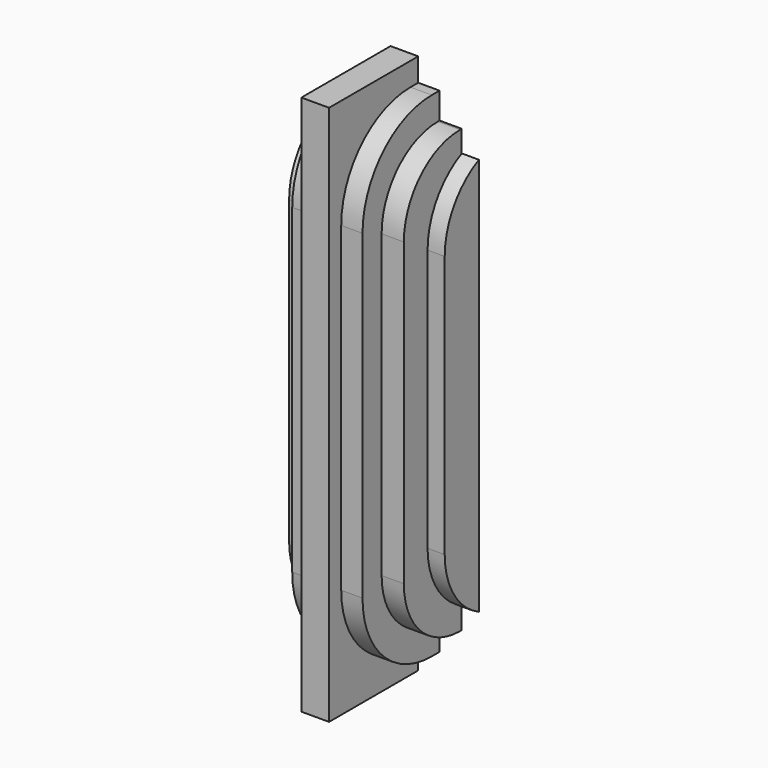
from build123d import *

# Parameters (mm, degrees)
F1_DEPTH      = 39.116
F2_DEPTH      = 33.782
F3_DEPTH      = 33.782
F4_DEPTH      = 25.4
F5_DEPTH      = 25.4
F0_W          = 6.0111228377
F0_H          = 69.8404787108
F6_DEPTH      = 14.986
F7_DEPTH      = 14.986
F8_T1_DEPTH   = 65.4734383573
F8_T6_DEPTH   = 124.9357538769
F10_R         = 24.6510518427
F11_R         = 24.6634
F12_R         = 30.3539071197
F14_T         = -2.54
F15_DEPTH     = 14.986
F16_T1_DEPTH  = 124.9268049826
F17_DEPTH     = 25.4
F18_R         = 24.6634
F19_DEPTH     = 33.782
F20_R         = 30.353
F21_DEPTH     = 39.116
F22_DEPTH     = 33.782
F23_DEPTH     = 25.4
F24_DEPTH     = 14.986
F25_T1_DEPTH  = 65.4689639101
F25_T6_DEPTH  = 124.9268049826
F26_R         = 24.6634
F27_R         = 30.353
F28_T         = 2.54
F28_T3_DEPTH  = 5.8166
F28_T5_DEPTH  = 110.6669781681
F28_T7_DEPTH  = 5.8289481573
F28_T9_DEPTH  = 8.509
F28_T11_DEPTH = 117.7830652202
F28_T13_DEPTH = 8.5080928803
F28_T15_DEPTH = 110.6546300108
F28_T17_DEPTH = 97.1928947849
F28_T19_DEPTH = 41.656
F28_T21_DEPTH = 9.7208591178
F28_T23_DEPTH = 10.414
F28_T25_DEPTH = 94.8683656752
F28_T27_DEPTH = 58.8910790502
F28_T29_DEPTH = 13.462
F28_T31_DEPTH = 55.3396631627
F28_T33_DEPTH = 15.494
F28_T35_DEPTH = 17.526
F28_T37_DEPTH = 48.595552503
F28_T39_DEPTH = 12.5542403813
F28_T41_DEPTH = 12.8764020893
F28_T43_DEPTH = 11.0911228377
F28_T45_DEPTH = 11.0911228377
F28_T47_DEPTH = 12.8764020893
F28_T49_DEPTH = 12.5542403813
F28_T51_DEPTH = 55.3273150054
F28_T54_ANGLE = 90.000000001
F28_T56_ANGLE = 90.000000001
F28_T58_ANGLE = 90.000000001
F28_T60_ANGLE = 90.000000001
F28_T62_ANGLE = 90.000000001
F28_T64_ANGLE = 90.000000001
F28_T66_ANGLE = 90.000000001
F28_T68_ANGLE = 90.000000001
F28_T70_ANGLE = 64.4309058664
F28_T72_ANGLE = 64.4270166015
F28_T74_ANGLE = 64.4309058664
F28_T76_ANGLE = 64.4270166015
F28_T78_ANGLE = 90.000000001
F28_T80_ANGLE = 90.000000001
F28_T82_ANGLE = 61.4663888849
F28_T84_ANGLE = 61.4663888848
F28_T86_ANGLE = 90.000000001
F28_T88_ANGLE = 90.000000001
F30_DEPTH     = 81.788


# Not quite as in the source:
# - a fillet or chamfer that OpenCascade refuses, or shapes differently, is made with other operations: its cross-section is extruded or revolved along the edge and cut away or added
# - two fillets or chamfers of one size are made in one step
# - a feature of the source that left no trace in its solid (it failed there, or was rolled back) is left out
# - a shell that OpenCascade refuses in one call is made with other operations: the cavity is built on its own and cut out


with BuildPart() as f1:
    # F0 (on Front) → F1 (new body)
    with BuildSketch(Plane.XZ):
        Polygon((4.8604295589, 33.4735736251), (0, 33.4735736251), (-4.8604295589, 33.4735736251), (-4.8604295589, 25.3101941198), (-4.8604295589, -61.3947920501), (4.8604295589, -61.3947920501), (4.8604295589, 25.3101941198), align=None)
    extrude(amount=F1_DEPTH)

    # F0 (on Front) → F2 (join)
    with BuildSketch(Plane.XZ):
        Polygon((-4.8604295589, -61.3947920501), (-4.8604295589, 25.3101941198), (-12.3346699402, 25.3101941198), (-12.3346699402, 16.0559229553), (-12.3346699402, -61.3947920501), align=None)
    extrude(amount=F2_DEPTH)

    # F0 (on Front) → F3 (join)
    with BuildSketch(Plane.XZ):
        Polygon((12.3346699402, 25.3101941198), (4.8604295589, 25.3101941198), (4.8604295589, -61.3947920501), (12.3346699402, -61.3947920501), (12.3346699402, 16.0559229553), align=None)
    extrude(amount=F3_DEPTH)

    # F0 (on Front) → F4 (join)
    with BuildSketch(Plane.XZ):
        Polygon((-20.1310720295, -61.3947920501), (-12.3346699402, -61.3947920501), (-12.3346699402, 16.0559229553), (-20.1310720295, 16.0559229553), (-20.1310720295, 8.4456866607), align=None)
    extrude(amount=F4_DEPTH)

    # F0 (on Front) → F5 (join)
    with BuildSketch(Plane.XZ):
        Polygon((12.3346699402, 16.0559229553), (12.3346699402, -61.3947920501), (20.1310720295, -61.3947920501), (20.1310720295, 8.4456866607), (20.1310720295, 16.0559229553), align=None)
    extrude(amount=F5_DEPTH)

    # F0 (on Front) → F6 (join)
    with BuildSketch(Plane.XZ):
        with Locations((-23.1366334483, -26.4745526947)):
            Rectangle(F0_W, F0_H)
    extrude(amount=F6_DEPTH)

    # F0 (on Front) → F7 (join)
    with BuildSketch(Plane.XZ):
        with Locations((23.1366334483, -26.4745526947)):
            Rectangle(F0_W, F0_H)
    extrude(amount=F7_DEPTH)

    # F8: fillet of radius 26.3680405282 on 1 edges, made by hand

    # F8_s2 → F8_t1 (cut)
    with BuildSketch(Plane.YZ.offset(20.1310720295)):
        with BuildLine():
            ThreePointArc((-14.986, -15.3392395471), (-10.9271018493, -1.2830762129), (0, 8.4456866607))
            Line((0, 8.4456866607), (-0.2276408106, 8.9213851849))
            ThreePointArc((-0.2276408106, 8.9213851849), (-7.493, 8.9730474713), (-14.986, 8.9730474713))
            Line((-14.986, 8.9730474713), (-15.5133608106, 8.4456866607))
            Line((-15.5133608106, 8.4456866607), (-15.5133608106, -15.3392395471))
            Line((-15.5133608106, -15.3392395471), (-14.986, -15.3392395471))
        make_face()
    extrude(amount=F8_T1_DEPTH, mode=Mode.SUBTRACT)


with BuildPart() as f8_tool4:
    # F8_s5 → F8_t6 (new body)
    with BuildSketch(Plane.YZ.offset(85.6045103867)):
        with BuildLine():
            ThreePointArc((-14.986, -15.3392395471), (-10.9271018493, -1.2830762129), (0, 8.4456866607))
            Line((0, 8.4456866607), (-0.2276408106, 8.9213851849))
            ThreePointArc((-0.2276408106, 8.9213851849), (-7.493, 8.9730474713), (-14.986, 8.9730474713))
            Line((-14.986, 8.9730474713), (-15.5133608106, 8.4456866607))
            Line((-15.5133608106, 8.4456866607), (-15.5133608106, -15.3392395471))
            Line((-15.5133608106, -15.3392395471), (-14.986, -15.3392395471))
        make_face()
    extrude(amount=-F8_T6_DEPTH)

    split(bisect_by=Plane.YZ.offset(-20.1310720295), keep=Keep.BOTTOM)


with BuildPart() as f1_1:
    add(f1.part)

    # F8_t3: cut F8_tool4
    add(f8_tool4.part, mode=Mode.SUBTRACT)

    # F10
    f10_edges = [f1_1.edges().sort_by_distance(p)[0] for p in [
        (16.232871, -25.4, 16.055923),
    ]]
    fillet(f10_edges, radius=F10_R)

    # F11
    f11_edges = [f1_1.edges().sort_by_distance(p)[0] for p in [
        (-16.232871, -25.4, 16.055923),
    ]]
    fillet(f11_edges, radius=F11_R)

    # F12
    f12_edges = [f1_1.edges().sort_by_distance(p)[0] for p in [
        (-8.59755, -33.782, 25.310194),
        (8.59755, -33.782, 25.310194),
    ]]
    fillet(f12_edges, radius=F12_R)

    # F14
    f14_openings = [f1_1.faces().sort_by_distance(p)[0] for p in [
        (0, 0, -20.12968),
    ]]
    offset(amount=F14_T, openings=f14_openings, kind=Kind.INTERSECTION)

    # F0 (on Front) → F15 (join)
    with BuildSketch(Plane.XZ):
        with Locations((-23.1366334483, -96.3150314055)):
            Rectangle(F0_W, F0_H)
    extrude(amount=F15_DEPTH)

    # F16: fillet of radius 26.3652 on 1 edges, made by hand

    # F16_s2 → F16_t1 (cut)
    with BuildSketch(Plane.YZ.offset(-85.6000359396)):
        with BuildLine():
            ThreePointArc((-14.986, -107.452134332), (-10.9270620679, -121.5075405374), (0, -131.235270761))
            Line((0, -131.235270761), (-14.986, -131.235270761))
            Line((-14.986, -131.235270761), (-14.986, -107.452134332))
        make_face()
    extrude(amount=F16_T1_DEPTH, mode=Mode.SUBTRACT)

    # F0 (on Front) → F17 (join)
    with BuildSketch(Plane.XZ):
        Polygon((-12.3346699402, -138.8455070555), (-12.3346699402, -61.3947920501), (-20.1310720295, -61.3947920501), (-20.1310720295, -131.235270761), (-20.1310720295, -138.8455070555), align=None)
    extrude(amount=F17_DEPTH)

    # F18
    f18_edges = [f1_1.edges().sort_by_distance(p)[0] for p in [
        (-16.232871, -25.4, -138.845507),
    ]]
    fillet(f18_edges, radius=F18_R)

    # F0 (on Front) → F19 (join)
    with BuildSketch(Plane.XZ):
        Polygon((-4.8604295589, -148.0997782201), (-4.8604295589, -61.3947920501), (-12.3346699402, -61.3947920501), (-12.3346699402, -138.8455070555), (-12.3346699402, -148.0997782201), align=None)
    extrude(amount=F19_DEPTH)

    # F20
    f20_edges = [f1_1.edges().sort_by_distance(p)[0] for p in [
        (-8.59755, -33.782, -148.099778),
    ]]
    fillet(f20_edges, radius=F20_R)

    # F0 (on Front) → F21 (join)
    with BuildSketch(Plane.XZ):
        Polygon((4.8604295589, -61.3947920501), (-4.8604295589, -61.3947920501), (-4.8604295589, -148.0997782201), (-4.8604295589, -156.2631577253), (0, -156.2631577253), (4.8604295589, -156.2631577253), (4.8604295589, -148.0997782201), align=None)
    extrude(amount=F21_DEPTH)

    # F0 (on Front) → F22 (join)
    with BuildSketch(Plane.XZ):
        Polygon((12.3346699402, -61.3947920501), (4.8604295589, -61.3947920501), (4.8604295589, -148.0997782201), (12.3346699402, -148.0997782201), (12.3346699402, -138.8455070555), align=None)
    extrude(amount=F22_DEPTH)

    # F0 (on Front) → F23 (join)
    with BuildSketch(Plane.XZ):
        Polygon((20.1310720295, -61.3947920501), (12.3346699402, -61.3947920501), (12.3346699402, -138.8455070555), (20.1310720295, -138.8455070555), (20.1310720295, -131.235270761), align=None)
    extrude(amount=F23_DEPTH)

    # F0 (on Front) → F24 (join)
    with BuildSketch(Plane.XZ):
        with Locations((23.1366334483, -96.3150314055)):
            Rectangle(F0_W, F0_H)
    extrude(amount=F24_DEPTH)

    # F25: fillet of radius 26.3652 on 1 edges, made by hand

    # F25_s2 → F25_t1 (cut)
    with BuildSketch(Plane.YZ.offset(20.1310720295)):
        with BuildLine():
            ThreePointArc((0, -131.235270761), (-10.9270620679, -121.5075405374), (-14.986, -107.452134332))
            Line((-14.986, -107.452134332), (-15.513304, -107.452134332))
            Line((-15.513304, -107.452134332), (-15.513304, -131.235270761))
            Line((-15.513304, -131.235270761), (-14.986, -131.762574761))
            ThreePointArc((-14.986, -131.762574761), (-7.493, -131.762574761), (-0.227584, -131.7109334895))
            Line((-0.227584, -131.7109334895), (0, -131.235270761))
        make_face()
    extrude(amount=F25_T1_DEPTH, mode=Mode.SUBTRACT)


with BuildPart() as f25_tool4:
    # F25_s5 → F25_t6 (new body)
    with BuildSketch(Plane.YZ.offset(-39.326769043)):
        with BuildLine():
            ThreePointArc((0, -131.235270761), (-10.9270620679, -121.5075405374), (-14.986, -107.452134332))
            Line((-14.986, -107.452134332), (-15.513304, -107.452134332))
            Line((-15.513304, -107.452134332), (-15.513304, -131.235270761))
            Line((-15.513304, -131.235270761), (-14.986, -131.762574761))
            ThreePointArc((-14.986, -131.762574761), (-7.493, -131.762574761), (-0.227584, -131.7109334895))
            Line((-0.227584, -131.7109334895), (0, -131.235270761))
        make_face()
    extrude(amount=F25_T6_DEPTH)

    split(bisect_by=Plane.YZ.offset(-20.1310720295), keep=Keep.BOTTOM)


with BuildPart() as f1_2:
    add(f1_1.part)

    # F25_t3: cut F25_tool4
    add(f25_tool4.part, mode=Mode.SUBTRACT)

    # F26
    f26_edges = [f1_2.edges().sort_by_distance(p)[0] for p in [
        (16.232871, -25.4, -138.845507),
    ]]
    fillet(f26_edges, radius=F26_R)

    # F27
    f27_edges = [f1_2.edges().sort_by_distance(p)[0] for p in [
        (8.59755, -33.782, -148.099778),
    ]]
    fillet(f27_edges, radius=F27_R)

    # F28: shell of thickness 2.54, made by hand


with BuildPart() as f28_core1:
    # F28_t2: copy of F1
    add(f1_2.part)

    # the walls: a layer under each face that stays
    f28_faces = [f28_core1.faces().sort_by_distance(p)[0] for p in [
        (12.3346699402, -28.1516666667, -119.1981161634),
        (8.5975497495, -1.7145, -148.0997782201),
        (8.5975497495, -24.8918121294, -139.2095903494),
        (8.5975497495, -33.782, -61.39524561),
        (16.2328709848, -0.3683, -138.8455070555),
        (8.5975497495, -24.8915464401, 16.41974056),
        (16.2328709848, -18.1762573871, -131.6217644426),
        (8.5975497495, -1.7140464401, 25.3101941198),
        (16.2328709848, -25.4, -61.3886179715),
        (16.2328709848, -18.1798740787, 8.8357970339),
        (16.2328709848, -0.3744740787, 16.0559229553),
        (4.8604295589, -36.322, -142.7105340574),
        (0, -19.558, 33.4735736251),
        (-4.8604295589, -36.322, 19.9209499572),
        (-8.5975497495, -1.7140464401, 25.3101941198),
        (-12.3346699402, -28.1516666667, -3.5914679368),
        (-16.2328709848, -0.3683, 16.0559229553),
        (-20.1310720295, -21.1666666667, -9.7609820465),
        (-23.1366334483, -10.9271018493, -1.2830762129),
        (-26.1421948671, -7.493, -61.3947920501),
        (-23.1366334483, -10.9270620679, -121.5075405375),
        (-16.2328709848, -0.3683, -138.8455070555),
        (-8.5975497495, -1.7145, -148.0997782201),
        (0, -19.558, -156.2631577253),
        (20.1310720295, -21.1666666667, -113.0286020537),
        (23.1366334483, -10.9270620679, -121.5075405375),
        (26.1421948671, -7.493, -61.3947920501),
        (23.1366334483, -10.9271018493, -1.2830762129),
        (0, -18.288, 30.9335736251),
        (2.3204295589, -30.48, 15.9688460126),
        (6.0575497495, -1.7140464401, 22.7701941198),
        (9.7946699402, -26.035, -45.2506276885),
        (13.6928709848, -0.3744740787, 13.5159229553),
        (17.5910720295, -19.05, -46.7930062159),
        (20.5966334483, -9.0995028513, -3.1621341354),
        (23.6021948671, -6.223, -26.6301076015),
        (0, -18.288, -58.8547920501),
        (-23.6021948671, -6.223, -26.6301076015),
        (-20.5966334483, -9.0995028513, -3.1621341354),
        (-17.5910720295, -19.05, 1.454137121),
        (-13.6928709848, -0.3683, 13.5159229553),
        (-9.7946699402, -26.035, 9.1660297582),
        (-6.0575497495, -1.7140464401, 22.7701941198),
        (-2.3204295589, -30.48, 15.9688460126),
        (0, -39.116, -61.3947920501),
        (-8.5975497495, -33.782, -61.39524561),
        (-8.5975497495, -24.8915464401, 16.41974056),
        (-8.5975497495, -24.8918121294, -139.2095903494),
        (-16.2328709848, -18.1762573871, -131.6217644426),
        (-16.2328709848, -18.1762573871, 8.8321803424),
        (-16.2328709848, -25.4, -61.3947920501),
        (-23.1366334483, -14.986, -61.3956869396),
        (23.1366334483, -14.986, -61.3956869395),
        (0, -36.576, -13.9606092125),
        (6.0575497495, -31.242, -31.949252525),
        (6.0575497495, -23.0954952159, 14.6236893357),
        (13.6928709848, -16.3838228544, 7.0397458097),
        (13.6928709848, -22.86, -33.7249604688),
        (20.5966334483, -12.446, -37.0970157986),
        (-20.5966334483, -12.446, -37.0970157986),
        (-13.6928709848, -22.86, -33.7311345474),
        (-6.0575497495, -31.242, -31.949252525),
        (-13.6928709848, -16.3802061629, 7.0361291182),
        (-6.0575497495, -23.0954952159, 14.6236893357),
    ]]
    thicken(f28_faces, amount=-F28_T, mode=Mode.SUBTRACT)

    # F28_s4 → F28_t3 (cut)
    with BuildSketch(Plane.XZ.offset(-2.54)):
        Polygon((12.3600699402, -138.8709070555), (9.7946699402, -138.8455070555), (9.7946699402, -136.3055070555), (12.3346699402, -136.3055070555), align=None)
        Polygon((-12.3600699402, -138.8709070555), (-9.7946699402, -138.8455070555), (-9.7946699402, -136.3055070555), (-12.3346699402, -136.3055070555), align=None)
        Polygon((-12.3600699402, 16.0813229553), (-9.7946699402, 16.0559229553), (-9.7946699402, 13.5159229553), (-12.3346699402, 13.5159229553), align=None)
        Polygon((-17.5656720295, 13.4905229553), (-20.1310720295, 13.5159229553), (-20.1310720295, 16.0559229553), (-17.5910720295, 16.0559229553), align=None)
    extrude(amount=F28_T3_DEPTH, mode=Mode.SUBTRACT)

    # F28_s6 → F28_t5 (cut)
    with BuildSketch(Plane.XY.offset(-116.7221070555)):
        Polygon((12.3600699402, -25.4254), (9.7946699402, -25.4), (9.7946699402, -22.86), (12.3346699402, -22.86), align=None)
    extrude(amount=F28_T5_DEPTH, mode=Mode.SUBTRACT)

    # F28_s8 → F28_t7 (cut)
    with BuildSketch(Plane.XZ.offset(-2.54)):
        Polygon((12.3600699402, 16.0813229553), (9.7946699402, 16.0559229553), (9.7946699402, 13.5159229553), (12.3346699402, 13.5159229553), align=None)
        Polygon((17.5656720295, 13.4905229553), (17.5910720295, 16.0559229553), (20.1310720295, 16.0559229553), (20.1310720295, 13.5159229553), align=None)
    extrude(amount=F28_T7_DEPTH, mode=Mode.SUBTRACT)

    # F28_s10 → F28_t9 (cut)
    with BuildSketch(Plane.XZ.offset(-2.54)):
        Polygon((4.8858295589, -148.1251782201), (4.8604295589, -145.5597782201), (2.3204295589, -145.5597782201), (2.3204295589, -148.0997782201), align=None)
        Polygon((-4.8858295589, -148.1251782201), (-2.3204295589, -148.0997782201), (-2.3204295589, -145.5597782201), (-4.8604295589, -145.5597782201), align=None)
    extrude(amount=F28_T9_DEPTH, mode=Mode.SUBTRACT)

    # F28_s12 → F28_t11 (cut)
    with BuildSketch(Plane.XY.offset(-120.2867782201)):
        Polygon((4.8858295589, -33.8074), (4.8604295589, -31.242), (2.3204295589, -31.242), (2.3204295589, -33.782), align=None)
        Polygon((-4.8858295589, -33.8074), (-2.3204295589, -33.782), (-2.3204295589, -31.242), (-4.8604295589, -31.242), align=None)
    extrude(amount=F28_T11_DEPTH, mode=Mode.SUBTRACT)

    # F28_s14 → F28_t13 (cut)
    with BuildSketch(Plane.XZ.offset(-2.54)):
        Polygon((4.8858295589, 25.3355941198), (4.8604295589, 22.7701941198), (2.3204295589, 22.7701941198), (2.3204295589, 25.3101941198), align=None)
        Polygon((-4.8858295589, 25.3355941198), (-2.3204295589, 25.3101941198), (-2.3204295589, 22.7701941198), (-4.8604295589, 22.7701941198), align=None)
        Polygon((9.7692699402, 22.7447941198), (9.7946699402, 25.3101941198), (12.3346699402, 25.3101941198), (12.3346699402, 22.7701941198), align=None)
        Polygon((-9.7692699402, 22.7447941198), (-12.3346699402, 22.7701941198), (-12.3346699402, 25.3101941198), (-9.7946699402, 25.3101941198), align=None)
    extrude(amount=F28_T13_DEPTH, mode=Mode.SUBTRACT)

    # F28_s16 → F28_t15 (cut)
    with BuildSketch(Plane.XY.offset(-116.7221070555)):
        Polygon((-12.3600699402, -25.4254), (-9.7946699402, -25.4), (-9.7946699402, -22.86), (-12.3346699402, -22.86), align=None)
    extrude(amount=F28_T15_DEPTH, mode=Mode.SUBTRACT)

    # F28_s18 → F28_t17 (cut)
    with BuildSketch(Plane.XY.offset(-109.992134332)):
        Polygon((-20.1564720295, -15.0114), (-17.5910720295, -14.986), (-17.5910720295, -12.446), (-20.1310720295, -12.446), align=None)
        Polygon((20.1564720295, -15.0114), (17.5910720295, -14.986), (17.5910720295, -12.446), (20.1310720295, -12.446), align=None)
    extrude(amount=F28_T17_DEPTH, mode=Mode.SUBTRACT)

    # F28_s20 → F28_t19 (cut)
    with BuildSketch(Plane.XZ.offset(-2.54)):
        Polygon((2.2950295589, 30.9081736251), (2.3204295589, 33.4735736251), (4.8604295589, 33.4735736251), (4.8604295589, 30.9335736251), align=None)
        Polygon((-2.2950295589, 30.9081736251), (-2.3204295589, 33.4735736251), (-4.8604295589, 33.4735736251), (-4.8604295589, 30.9335736251), align=None)
    extrude(amount=F28_T19_DEPTH, mode=Mode.SUBTRACT)

    # F28_s22 → F28_t21 (cut)
    with BuildSketch(Plane.YZ.offset(-4.8604295589)):
        Polygon((-36.5506, 30.9081736251), (-36.576, 33.4735736251), (-39.116, 33.4735736251), (-39.116, 30.9335736251), align=None)
        Polygon((-36.5506, -58.8293920501), (-36.576, -61.3947920501), (-39.116, -61.3947920501), (-39.116, -58.8547920501), align=None)
    extrude(amount=F28_T21_DEPTH, mode=Mode.SUBTRACT)

    # F28_s24 → F28_t23 (cut)
    with BuildSketch(Plane.XZ.offset(28.702)):
        Polygon((2.2950295589, -58.8293920501), (4.8604295589, -58.8547920501), (4.8604295589, -61.3947920501), (2.3204295589, -61.3947920501), align=None)
        Polygon((-2.2950295589, -58.8293920501), (-2.3204295589, -61.3947920501), (-4.8604295589, -61.3947920501), (-4.8604295589, -58.8547920501), align=None)
    extrude(amount=F28_T23_DEPTH, mode=Mode.SUBTRACT)

    # F28_s26 → F28_t25 (cut)
    with BuildSketch(Plane.XY.offset(-61.3947920501)):
        Polygon((2.2950295589, -36.5506), (4.8604295589, -36.576), (4.8604295589, -39.116), (2.3204295589, -39.116), align=None)
        Polygon((-2.2950295589, -36.5506), (-4.8604295589, -36.576), (-4.8604295589, -39.116), (-2.3204295589, -39.116), align=None)
    extrude(amount=F28_T25_DEPTH, mode=Mode.SUBTRACT)

    # F28_s28 → F28_t27 (cut)
    with BuildSketch(Plane.XY.offset(-61.3947920501)):
        Polygon((9.7692699402, -31.2166), (12.3346699402, -31.242), (12.3346699402, -33.782), (9.7946699402, -33.782), align=None)
        Polygon((-9.7692699402, -31.2166), (-12.3346699402, -31.242), (-12.3346699402, -33.782), (-9.7946699402, -33.782), align=None)
    extrude(amount=F28_T27_DEPTH, mode=Mode.SUBTRACT)

    # F28_s30 → F28_t29 (cut)
    with BuildSketch(Plane.XZ.offset(20.32)):
        Polygon((9.7692699402, -58.8293920501), (12.3346699402, -58.8547920501), (12.3346699402, -61.3947920501), (9.7946699402, -61.3947920501), align=None)
        Polygon((-9.7692699402, -58.8293920501), (-9.7946699402, -61.3947920501), (-12.3346699402, -61.3947920501), (-12.3346699402, -58.8547920501), align=None)
    extrude(amount=F28_T29_DEPTH, mode=Mode.SUBTRACT)

    # F28_s32 → F28_t31 (cut)
    with BuildSketch(Plane.XY.offset(-61.3947920501)):
        Polygon((17.5656720295, -22.8346), (20.1310720295, -22.86), (20.1310720295, -25.4), (17.5910720295, -25.4), align=None)
    extrude(amount=F28_T31_DEPTH, mode=Mode.SUBTRACT)

    # F28_s34 → F28_t33 (cut)
    with BuildSketch(Plane.XZ.offset(9.906)):
        Polygon((17.5656720295, -58.8293920501), (20.1310720295, -58.8547920501), (20.1310720295, -61.3947920501), (17.5910720295, -61.3947920501), align=None)
        Polygon((-17.5656720295, -58.8293920501), (-17.5910720295, -61.3947920501), (-20.1310720295, -61.3947920501), (-20.1310720295, -58.8547920501), align=None)
    extrude(amount=F28_T33_DEPTH, mode=Mode.SUBTRACT)

    # F28_s36 → F28_t35 (cut)
    with BuildSketch(Plane.XZ.offset(-2.54)):
        Polygon((23.5767948671, -58.8293920501), (26.1421948671, -58.8547920501), (26.1421948671, -61.3947920501), (23.6021948671, -61.3947920501), align=None)
        Polygon((-23.5767948671, -58.8293920501), (-23.6021948671, -61.3947920501), (-26.1421948671, -61.3947920501), (-26.1421948671, -58.8547920501), align=None)
    extrude(amount=F28_T35_DEPTH, mode=Mode.SUBTRACT)

    # F28_s38 → F28_t37 (cut)
    with BuildSketch(Plane.XY.offset(-61.3947920501)):
        Polygon((23.5767948671, -12.4206), (26.1421948671, -12.446), (26.1421948671, -14.986), (23.6021948671, -14.986), align=None)
        Polygon((-23.5767948671, -12.4206), (-26.1421948671, -12.446), (-26.1421948671, -14.986), (-23.6021948671, -14.986), align=None)
    extrude(amount=F28_T37_DEPTH, mode=Mode.SUBTRACT)

    # F28_s40 → F28_t39 (cut)
    with BuildSketch(Plane.YZ.offset(-0.2195704411)):
        Polygon((-31.2166, -58.8293920501), (-31.242, -61.3947920501), (-33.782, -61.3947920501), (-33.782, -58.8547920501), align=None)
    extrude(amount=F28_T39_DEPTH, mode=Mode.SUBTRACT)

    # F28_s42 → F28_t41 (cut)
    with BuildSketch(Plane.YZ.offset(7.2546699402)):
        Polygon((-22.8346, -58.8293920501), (-22.86, -61.3947920501), (-25.4, -61.3947920501), (-25.4, -58.8547920501), align=None)
    extrude(amount=F28_T41_DEPTH, mode=Mode.SUBTRACT)

    # F28_s44 → F28_t43 (cut)
    with BuildSketch(Plane.YZ.offset(15.0510720295)):
        Polygon((-12.4206, -58.8293920501), (-12.446, -61.3947920501), (-14.986, -61.3947920501), (-14.986, -58.8547920501), align=None)
    extrude(amount=F28_T43_DEPTH, mode=Mode.SUBTRACT)

    # F28_s46 → F28_t45 (cut)
    with BuildSketch(Plane.YZ.offset(-26.1421948671)):
        Polygon((-12.4206, -58.8293920501), (-12.446, -61.3947920501), (-14.986, -61.3947920501), (-14.986, -58.8547920501), align=None)
    extrude(amount=F28_T45_DEPTH, mode=Mode.SUBTRACT)

    # F28_s48 → F28_t47 (cut)
    with BuildSketch(Plane.YZ.offset(-20.1310720295)):
        Polygon((-22.8346, -58.8293920501), (-22.86, -61.3947920501), (-25.4, -61.3947920501), (-25.4, -58.8547920501), align=None)
    extrude(amount=F28_T47_DEPTH, mode=Mode.SUBTRACT)

    # F28_s50 → F28_t49 (cut)
    with BuildSketch(Plane.YZ.offset(-12.3346699402)):
        Polygon((-31.2166, -58.8293920501), (-31.242, -61.3947920501), (-33.782, -61.3947920501), (-33.782, -58.8547920501), align=None)
    extrude(amount=F28_T49_DEPTH, mode=Mode.SUBTRACT)

    # F28_s52 → F28_t51 (cut)
    with BuildSketch(Plane.XY.offset(-61.3947920501)):
        Polygon((-17.5656720295, -22.8346), (-20.1310720295, -22.86), (-20.1310720295, -25.4), (-17.5910720295, -25.4), align=None)
    extrude(amount=F28_T51_DEPTH, mode=Mode.SUBTRACT)

    # F28_s53 → F28_t54 (revolve, cut)
    with BuildSketch(Plane.XZ.offset(0.7366)):
        Polygon((12.3600699402, -138.8709070555), (9.7946699402, -138.8455070555), (9.7946699402, -136.3055070555), (12.3346699402, -136.3055070555), align=None)
    revolve(axis=Axis((12.3346699402, -0.7366, -114.1821070555), (-1, 0, 0)), revolution_arc=F28_T54_ANGLE, mode=Mode.SUBTRACT)

    # F28_s55 → F28_t56 (revolve, cut)
    with BuildSketch(Plane.XZ.offset(0.7489481573)):
        Polygon((12.3600699402, 16.0813229553), (9.7946699402, 16.0559229553), (9.7946699402, 13.5159229553), (12.3346699402, 13.5159229553), align=None)
    revolve(axis=Axis((12.3346699402, -0.7489481573, -8.5951288874), (1, 0, 0)), revolution_arc=F28_T56_ANGLE, mode=Mode.SUBTRACT)

    # F28_s57 → F28_t58 (revolve, cut)
    with BuildSketch(Plane.XZ.offset(3.429)):
        Polygon((4.8858295589, -148.1251782201), (4.8604295589, -145.5597782201), (2.3204295589, -145.5597782201), (2.3204295589, -148.0997782201), align=None)
    revolve(axis=Axis((4.8604295589, -3.429, -117.7467782201), (-1, 0, 0)), revolution_arc=F28_T58_ANGLE, mode=Mode.SUBTRACT)

    # F28_s59 → F28_t60 (revolve, cut)
    with BuildSketch(Plane.XZ.offset(3.4280928803)):
        Polygon((4.8858295589, 25.3355941198), (4.8604295589, 22.7701941198), (2.3204295589, 22.7701941198), (2.3204295589, 25.3101941198), align=None)
    revolve(axis=Axis((4.8604295589, -3.4280928803, -5.0437129999), (1, 0, 0)), revolution_arc=F28_T60_ANGLE, mode=Mode.SUBTRACT)

    # F28_s61 → F28_t62 (revolve, cut)
    with BuildSketch(Plane.XZ.offset(3.4280928803)):
        Polygon((-4.8858295589, 25.3355941198), (-2.3204295589, 25.3101941198), (-2.3204295589, 22.7701941198), (-4.8604295589, 22.7701941198), align=None)
    revolve(axis=Axis((-4.8604295589, -3.4280928803, -5.0437129999), (1, 0, 0)), revolution_arc=F28_T62_ANGLE, mode=Mode.SUBTRACT)

    # F28_s63 → F28_t64 (revolve, cut)
    with BuildSketch(Plane.XY.offset(-117.7467782201)):
        Polygon((-4.8858295589, -33.8074), (-2.3204295589, -33.782), (-2.3204295589, -31.242), (-4.8604295589, -31.242), align=None)
    revolve(axis=Axis((-4.8604295589, -3.429, -117.7467782201), (1, 0, 0)), revolution_arc=F28_T64_ANGLE, mode=Mode.SUBTRACT)

    # F28_s65 → F28_t66 (revolve, cut)
    with BuildSketch(Plane.XY.offset(-114.1821070555)):
        Polygon((-12.3600699402, -25.4254), (-9.7946699402, -25.4), (-9.7946699402, -22.86), (-12.3346699402, -22.86), align=None)
    revolve(axis=Axis((-12.3346699402, -0.7366, -114.1821070555), (1, 0, 0)), revolution_arc=F28_T66_ANGLE, mode=Mode.SUBTRACT)

    # F28_s67 → F28_t68 (revolve, cut)
    with BuildSketch(Plane.XY.offset(-8.6074770447)):
        Polygon((-12.3600699402, -25.4254), (-9.7946699402, -25.4), (-9.7946699402, -22.86), (-12.3346699402, -22.86), align=None)
    revolve(axis=Axis((-12.3346699402, -0.7366, -8.6074770447), (-1, 0, 0)), revolution_arc=F28_T68_ANGLE, mode=Mode.SUBTRACT)

    # F28_s69 → F28_t70 (revolve, cut)
    with BuildSketch(Plane(origin=(0, 51.0939277003, -24.4462299504), x_dir=(1, 0, 0), z_dir=(0, 0.9020654662, -0.4315992293))):
        Polygon((-20.1564720295, 118.4082056986), (-17.5910720295, 118.3828056986), (-17.5910720295, 115.8428056986), (-20.1310720295, 115.8428056986), align=None)
    revolve(axis=Axis((-20.1310720295, 11.3792, -107.452134332), (-1, 0, 0)), revolution_arc=F28_T70_ANGLE, mode=Mode.SUBTRACT)

    # F28_s71 → F28_t72 (revolve, cut)
    with BuildSketch(Plane(origin=(0, 3.2885252878, 1.5736911595), x_dir=(1, 0, 0), z_dir=(0, 0.9020361669, 0.4316604609))):
        Polygon((-20.1564720295, -7.6437148226), (-17.5910720295, -7.6183148226), (-17.5910720295, -5.0783148226), (-20.1310720295, -5.0783148226), align=None)
    revolve(axis=Axis((-20.1310720295, 11.3820405281, -15.3392395471), (1, 0, 0)), revolution_arc=F28_T72_ANGLE, mode=Mode.SUBTRACT)

    # F28_s73 → F28_t74 (revolve, cut)
    with BuildSketch(Plane(origin=(0, 51.0939277003, -24.4462299504), x_dir=(1, 0, 0), z_dir=(0, 0.9020654662, -0.4315992293))):
        Polygon((20.1564720295, 118.4082056986), (17.5910720295, 118.3828056986), (17.5910720295, 115.8428056986), (20.1310720295, 115.8428056986), align=None)
    revolve(axis=Axis((20.1310720295, 11.3792, -107.452134332), (-1, 0, 0)), revolution_arc=F28_T74_ANGLE, mode=Mode.SUBTRACT)

    # F28_s75 → F28_t76 (revolve, cut)
    with BuildSketch(Plane.XY.offset(-15.3392395471)):
        Polygon((20.1564720295, -15.0114), (17.5910720295, -14.986), (17.5910720295, -12.446), (20.1310720295, -12.446), align=None)
    revolve(axis=Axis((20.1310720295, 11.3820405281, -15.3392395471), (-1, 0, 0)), revolution_arc=F28_T76_ANGLE, mode=Mode.SUBTRACT)

    # F28_s77 → F28_t78 (revolve, cut)
    with BuildSketch(Plane.XY.offset(-5.0437129999)):
        Polygon((9.7692699402, -31.2166), (12.3346699402, -31.242), (12.3346699402, -33.782), (9.7946699402, -33.782), align=None)
    revolve(axis=Axis((9.7946699402, -3.4280928803, -5.0437129999), (-1, 0, 0)), revolution_arc=F28_T78_ANGLE, mode=Mode.SUBTRACT)

    # F28_s79 → F28_t80 (revolve, cut)
    with BuildSketch(Plane.XY.offset(-8.5951288874)):
        Polygon((17.5656720295, -22.8346), (20.1310720295, -22.86), (20.1310720295, -25.4), (17.5910720295, -25.4), align=None)
    revolve(axis=Axis((17.5910720295, -0.7489481573, -8.5951288874), (-1, 0, 0)), revolution_arc=F28_T80_ANGLE, mode=Mode.SUBTRACT)

    # F28_s81 → F28_t82 (revolve, cut)
    with BuildSketch(Plane.XY.offset(-15.3392395471)):
        Polygon((23.5767948671, -12.4206), (23.6021948671, -14.986), (26.1421948671, -14.986), (26.1421948671, -12.446), align=None)
    revolve(axis=Axis((23.6021948671, 11.3820405281, -15.3392395471), (-1, 0, 0)), revolution_arc=F28_T82_ANGLE, mode=Mode.SUBTRACT)

    # F28_s83 → F28_t84 (revolve, cut)
    with BuildSketch(Plane(origin=(0, 2.3477893158, 1.2765294507), x_dir=(1, 0, 0), z_dir=(0, 0.8785370484, 0.4776742139))):
        Polygon((-23.5767948671, -4.8896430302), (-26.1421948671, -4.9150430302), (-26.1421948671, -7.4550430302), (-23.6021948671, -7.4550430302), align=None)
    revolve(axis=Axis((-23.6021948671, 11.3820405281, -15.3392395471), (1, 0, 0)), revolution_arc=F28_T84_ANGLE, mode=Mode.SUBTRACT)

    # F28_s85 → F28_t86 (revolve, cut)
    with BuildSketch(Plane.XY.offset(-8.6074770447)):
        Polygon((-17.5656720295, -22.8346), (-20.1310720295, -22.86), (-20.1310720295, -25.4), (-17.5910720295, -25.4), align=None)
    revolve(axis=Axis((-17.5910720295, -0.7366, -8.6074770447), (-1, 0, 0)), revolution_arc=F28_T86_ANGLE, mode=Mode.SUBTRACT)

    # F28_s87 → F28_t88 (revolve, cut)
    with BuildSketch(Plane.XY.offset(-5.0437129999)):
        Polygon((-9.7692699402, -31.2166), (-12.3346699402, -31.242), (-12.3346699402, -33.782), (-9.7946699402, -33.782), align=None)
    revolve(axis=Axis((-9.7946699402, -3.4280928803, -5.0437129999), (-1, 0, 0)), revolution_arc=F28_T88_ANGLE, mode=Mode.SUBTRACT)


with BuildPart() as f1_3:
    add(f1_2.part)

    # what is left inside the walls is the cavity
    f28_cavity = [f28_core1.part.solids().sort_by_distance(p)[0] for p in [
        (0, -0.0254, -122.947036),
    ]]
    add(f28_cavity, mode=Mode.SUBTRACT)

    # F29 (on Top) → F30 (cut)
    with BuildSketch(Plane.XY):
        with BuildLine():
            Line((-7.62, 3.1624301337), (-7.62, -4.8556555994))
            ThreePointArc((-7.62, -4.8556555994), (0, -12.4756555994), (7.62, -4.8556555994))
            Line((7.62, -4.8556555994), (7.62, 3.1624301337))
            Line((7.62, 3.1624301337), (-7.62, 3.1624301337))
        make_face()
    extrude(amount=-F30_DEPTH, mode=Mode.SUBTRACT)


solid = f1_3.part
